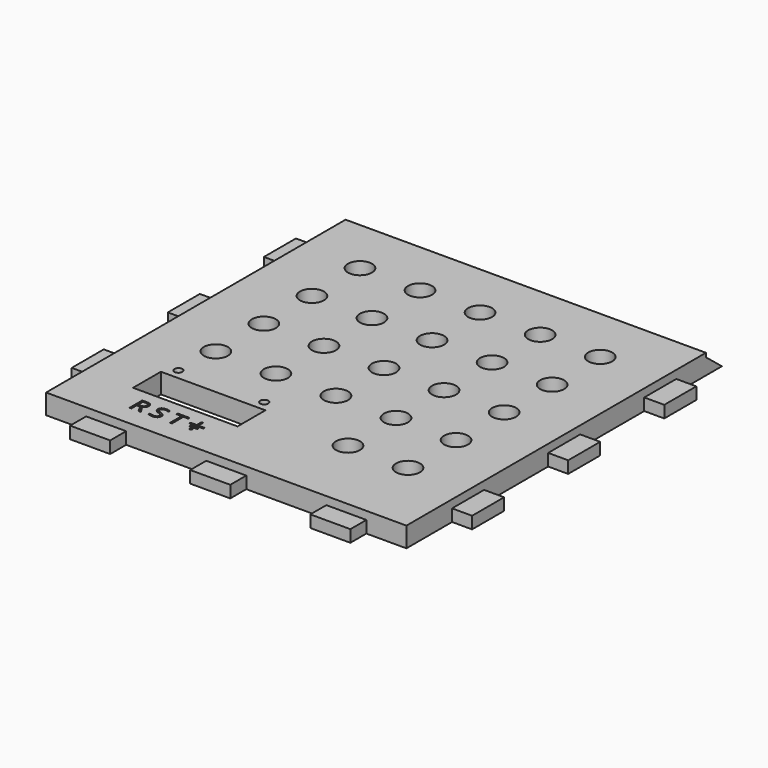
from build123d import *

# Parameters (mm, degrees)
F0_W          = 90
F0_H          = 98.5
F1_DEPTH      = 5
F3_DEPTH      = 100
F4_W          = 10
F4_H          = 3
F5_DEPTH      = 95
F5_DEPTH_BACK = 5
F6_W          = 10
F6_H          = 3
F7_DEPTH      = 5
F8_W          = 26.1
F8_H          = 8.7
F8_R          = 1
F9_DEPTH      = 25
F10_R         = 0.3
F10_W         = 2
F10_H         = 0.4
F10_W_2       = 0.4
F10_H_2       = 1.5
F10_TEXT_SIZE = 5.5555555556
F11_DEPTH     = 0.5
F12_R         = 3
F13_DEPTH     = 25
F15_DEPTH     = 2


# Not quite as in the source:
# - Text() gives the source's letters only with a copy of the font that has no kerning and outlines rounded to 1/6400 em; it was checked with that copy


with BuildPart() as f1:
    # F0 (on Top) → F1 (new body)
    with BuildSketch(Plane.XY):
        Rectangle(F0_W, F0_H)
    extrude(amount=F1_DEPTH)

    # F2 (on face) → F3 (cut)
    with BuildSketch(Plane.YZ.offset(45)):
        Polygon((49.25, 0), (49.25, 5), (44.25, 5), (44.25, 4), align=None)
    extrude(amount=-F3_DEPTH, mode=Mode.SUBTRACT)

    # F4 (on face) → F5 (join, two sides)
    with BuildSketch(Plane.YZ.offset(45)) as f5_sk:
        with Locations((0, 1.5)):
            Rectangle(F4_W, F4_H)
        with Locations((30, 1.5)):
            Rectangle(F4_W, F4_H)
        with Locations((-30, 1.5)):
            Rectangle(F4_W, F4_H)
    extrude(amount=-F5_DEPTH)
    extrude(f5_sk.sketch, amount=F5_DEPTH_BACK)

    # F6 (on face) → F7 (join)
    with BuildSketch(Plane.XZ.offset(49.25)):
        with Locations((-30, 1.5)):
            Rectangle(F6_W, F6_H)
        with Locations((0, 1.5)):
            Rectangle(F6_W, F6_H)
        with Locations((30, 1.5)):
            Rectangle(F6_W, F6_H)
    extrude(amount=F7_DEPTH)

    # F8 (on face) → F9 (cut)
    with BuildSketch(Plane.XY.offset(5)):
        with Locations((-19.95, -32.75)):
            Rectangle(F8_W, F8_H)
        with Locations((-30.665, -25.85)):
            Circle(F8_R)
        with Locations((-9.235, -25.85)):
            Circle(F8_R)
    extrude(amount=-F9_DEPTH, mode=Mode.SUBTRACT)

    # F10 (on face) → F11 (cut)
    with BuildSketch(Plane.XY.offset(5)):
        with Locations((-13.2973958333, -43.65)):
            Circle(F10_R)
        with Locations((-13.2973958333, -42.7)):
            Rectangle(F10_W, F10_H)
        Polygon((-13.4973958333, -41.6), (-15.0473958333, -41.6), (-15.0473958333, -42), (-11.5473958333, -42), (-11.5473958333, -41.6), (-13.0973958333, -41.6), align=None)
        with Locations((-13.2973958333, -40.85)):
            Rectangle(F10_W_2, F10_H_2)
        with Locations((-28.8, -44.1)):
            Text('R S T', F10_TEXT_SIZE, font='Open Sans', text_align=(TextAlign.LEFT, TextAlign.BOTTOM))
    extrude(amount=-F11_DEPTH, mode=Mode.SUBTRACT)

    # F12 (on face) → F13 (cut)
    with BuildSketch(Plane.XY.offset(5)):
        with Locations((-30, 30)):
            Circle(F12_R)
        with Locations((-30, 15)):
            Circle(F12_R)
        with Locations((-30, 0)):
            Circle(F12_R)
        with Locations((-30, -15)):
            Circle(F12_R)
        with Locations((-15, 30)):
            Circle(F12_R)
        with Locations((-15, 15)):
            Circle(F12_R)
        with Locations((-15, 0)):
            Circle(F12_R)
        with Locations((-15, -15)):
            Circle(F12_R)
        with Locations((0, 30)):
            Circle(F12_R)
        with Locations((0, 15)):
            Circle(F12_R)
        Circle(F12_R)
        with Locations((0, -15)):
            Circle(F12_R)
        with Locations((15, 30)):
            Circle(F12_R)
        with Locations((15, 15)):
            Circle(F12_R)
        with Locations((15, 0)):
            Circle(F12_R)
        with Locations((15, -15)):
            Circle(F12_R)
        with Locations((30, 30)):
            Circle(F12_R)
        with Locations((30, 15)):
            Circle(F12_R)
        with Locations((30, 0)):
            Circle(F12_R)
        with Locations((30, -15)):
            Circle(F12_R)
        with Locations((30, -30)):
            Circle(F12_R)
        with Locations((15, -30)):
            Circle(F12_R)
    extrude(amount=-F13_DEPTH, mode=Mode.SUBTRACT)

    # F14 (on face) → F15 (cut)
    with BuildSketch(Plane(origin=(0, 0, 0), x_dir=(1, 0, 0), z_dir=(0, 0, -1))):
        Polygon((-31.8197005384, 23.85), (-29.5102994616, 23.85), (-28.3555989232, 25.85), (-29.5102994616, 27.85), (-31.8197005384, 27.85), (-32.9744010768, 25.85), align=None)
        Polygon((-10.3897005384, 23.85), (-8.0802994616, 23.85), (-6.9255989232, 25.85), (-8.0802994616, 27.85), (-10.3897005384, 27.85), (-11.5444010768, 25.85), align=None)
    extrude(amount=-F15_DEPTH, mode=Mode.SUBTRACT)


solid = f1.part
